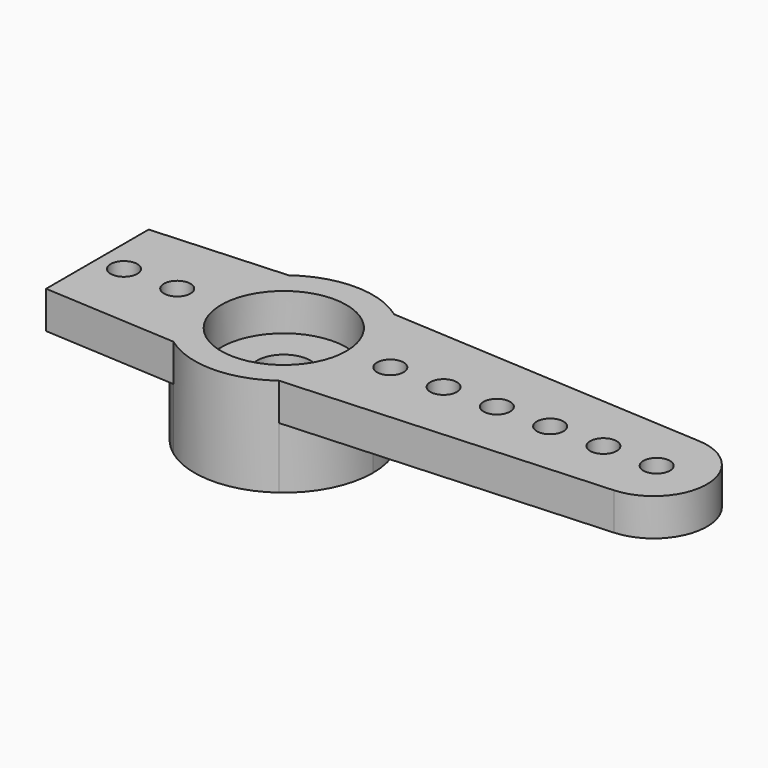
from build123d import *

# Parameters (mm, degrees)
F0_R     = 2.35
F0_R_2   = 0.5
F1_DEPTH = 1.4
F2_R     = 2.35
F2_R_2   = 1
F3_DEPTH = 2.3
F4_R     = 2.35
F4_R_2   = 1
F5_DEPTH = 1.8


with BuildPart() as f1:
    # F0 (on Top) → F1 (new body)
    with BuildSketch(Plane.XY):
        with BuildLine():
            ThreePointArc((1.9830532015, -2.7), (2.9887897404, -1.5131542841), (3.35, 0))
            ThreePointArc((3.35, 0), (2.9887897404, 1.5131542841), (1.9830532015, 2.7))
            ThreePointArc((1.9830532015, 2.7), (0, 3.35), (-1.9830532015, 2.7))
            ThreePointArc((-1.9830532015, 2.7), (-3.35, 0), (-1.9830532015, -2.7))
            ThreePointArc((-1.9830532015, -2.7), (0, -3.35), (1.9830532015, -2.7))
        make_face()
        Circle(F0_R, mode=Mode.SUBTRACT)
        with BuildLine():
            ThreePointArc((1.9830532015, 2.7), (2.9887897404, 1.5131542841), (3.35, 0))
            ThreePointArc((3.35, 0), (2.9887897404, -1.5131542841), (1.9830532015, -2.7))
            Line((1.9830532015, -2.7), (14, -2))
            ThreePointArc((14, -2), (15.886888175, 0), (14, 2))
            Line((14, 2), (1.9830532015, 2.7))
        make_face()
        with Locations((4, 0)):
            Circle(F0_R_2, mode=Mode.SUBTRACT)
        with Locations((6, 0)):
            Circle(F0_R_2, mode=Mode.SUBTRACT)
        with Locations((8, 0)):
            Circle(F0_R_2, mode=Mode.SUBTRACT)
        with Locations((10, 0)):
            Circle(F0_R_2, mode=Mode.SUBTRACT)
        with Locations((12, 0)):
            Circle(F0_R_2, mode=Mode.SUBTRACT)
        with Locations((14, 0)):
            Circle(F0_R_2, mode=Mode.SUBTRACT)
        with BuildLine():
            ThreePointArc((-1.9830532015, -2.7), (-3.35, 0), (-1.9830532015, 2.7))
            Line((-1.9830532015, 2.7), (-6.9970610693, 2.4079286805))
            Line((-6.9970610693, 2.4079286805), (-6.9970610693, -2.4079286805))
            Line((-6.9970610693, -2.4079286805), (-1.9830532015, -2.7))
        make_face()
        with Locations((-6, 0)):
            Circle(F0_R_2, mode=Mode.SUBTRACT)
        with Locations((-4, 0)):
            Circle(F0_R_2, mode=Mode.SUBTRACT)
    extrude(amount=F1_DEPTH)

    # F2 (on face) → F3 (join)
    with BuildSketch(Plane(origin=(0, 0, 0), x_dir=(1, 0, 0), z_dir=(0, 0, -1))):
        with BuildLine():
            ThreePointArc((1.9830532015, -2.7), (2.9887897404, -1.5131542841), (3.35, 0))
            ThreePointArc((3.35, 0), (2.9887897404, 1.5131542841), (1.9830532015, 2.7))
            ThreePointArc((1.9830532015, 2.7), (0, 3.35), (-1.9830532015, 2.7))
            ThreePointArc((-1.9830532015, 2.7), (-3.35, 0), (-1.9830532015, -2.7))
            ThreePointArc((-1.9830532015, -2.7), (0, -3.35), (1.9830532015, -2.7))
        make_face()
        Circle(F2_R, mode=Mode.SUBTRACT)
        Circle(F2_R)
        Circle(F2_R_2, mode=Mode.SUBTRACT)
    extrude(amount=F3_DEPTH)

    # F4 (on face) → F5 (cut)
    with BuildSketch(Plane(origin=(0, 0, -2.3), x_dir=(1, 0, 0), z_dir=(0, 0, -1))):
        Circle(F4_R)
        Circle(F4_R_2, mode=Mode.SUBTRACT)
    extrude(amount=-F5_DEPTH, mode=Mode.SUBTRACT)


solid = f1.part
